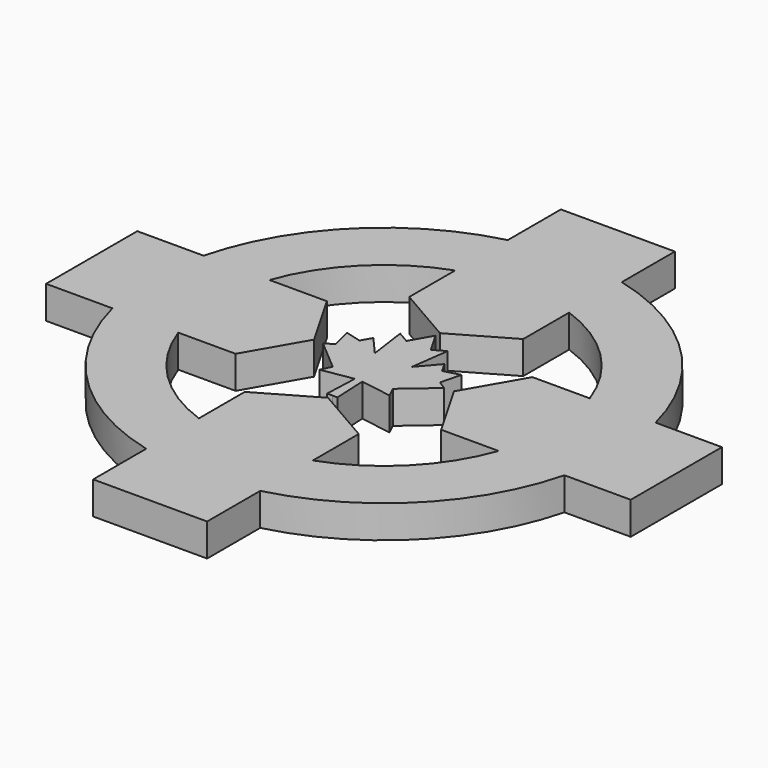
from build123d import *

# Parameters (mm, degrees)
F1_DEPTH = 5


with BuildPart() as f1:
    # F0 (on Top) → F1 (new body)
    with BuildSketch(Plane.XY):
        with BuildLine():
            Line((-8.7284976617, 44.7745621204), (-8.7284976617, 34.6139920432))
            ThreePointArc((-8.7284976617, 34.6139920432), (-4.3977485861, 35.4256252446), (0, 35.6975505686))
            Line((0, 35.6975505686), (0, 44.7745621204))
            Line((0, 44.7745621204), (-8.7284976617, 44.7745621204))
        make_face()
        with BuildLine():
            Line((0, 44.7745621204), (0, 35.6975505686))
            ThreePointArc((0, 35.6975505686), (4.3977485861, 35.4256252446), (8.7284976617, 34.6139920432))
            Line((8.7284976617, 34.6139920432), (8.7284976617, 44.7745621204))
            Line((8.7284976617, 44.7745621204), (0, 44.7745621204))
        make_face()
        with BuildLine():
            ThreePointArc((8.7284976617, 34.6139920432), (4.3977485861, 35.4256252446), (0, 35.6975505686))
            Line((0, 35.6975505686), (0, 26.0385947902))
            ThreePointArc((0, 26.0385947902), (4.4287789528, 25.6591959273), (8.7284976616, 24.5320555033))
            Line((8.7284976617, 24.5320555033), (8.7284976617, 34.6139920432))
        make_face()
        with BuildLine():
            ThreePointArc((0, 35.6975505686), (-4.3977485861, 35.4256252446), (-8.7284976617, 34.6139920432))
            Line((-8.7284976617, 34.6139920432), (-8.7284976617, 24.5320555033))
            ThreePointArc((-8.7284976616, 24.5320555033), (-4.4287789528, 25.6591959273), (0, 26.0385947902))
            Line((0, 26.0385947902), (0, 35.6975505686))
        make_face()
        with BuildLine():
            ThreePointArc((0, 26.0385947902), (-4.4287789528, 25.6591959273), (-8.7284976616, 24.5320555033))
            Line((-8.7284976617, 24.5320555033), (-8.7284976617, 15.7472789288))
            Line((-8.7284976617, 15.7472789288), (0, 10.7151791453))
            Line((0, 10.7151791453), (0, 26.0385947902))
        make_face()
        with BuildLine():
            ThreePointArc((8.7284976616, 24.5320555033), (4.4287789528, 25.6591959273), (0, 26.0385947902))
            Line((0, 26.0385947902), (0, 10.7151791453))
            Line((0, 10.7151791453), (8.7284976617, 15.7472789288))
            Line((8.7284976617, 15.7472789288), (8.7284976617, 24.5320555033))
        make_face()
        with BuildLine():
            Line((15.7472789288, -8.7284976617), (24.5320555033, -8.7284976617))
            ThreePointArc((24.5320555033, -8.7284976617), (25.6591959273, -4.4287789528), (26.0385947902, 0))
            Line((26.0385947902, 0), (10.7151791453, 0))
            Line((10.7151791453, 0), (15.7472789288, -8.7284976617))
        make_face()
        with BuildLine():
            ThreePointArc((26.0385947902, 0), (25.6591959273, 4.4287789528), (24.5320555033, 8.7284976616))
            Line((24.5320555033, 8.7284976617), (15.7472789288, 8.7284976617))
            Line((15.7472789288, 8.7284976617), (10.7151791453, 0))
            Line((10.7151791453, 0), (26.0385947902, 0))
        make_face()
        with BuildLine():
            ThreePointArc((35.6975505686, 0), (35.4256252446, 4.3977485861), (34.6139920432, 8.7284976616))
            Line((34.6139920432, 8.7284976617), (24.5320555033, 8.7284976617))
            ThreePointArc((24.5320555033, 8.7284976616), (25.6591959273, 4.4287789528), (26.0385947902, 0))
            Line((26.0385947902, 0), (35.6975505686, 0))
        make_face()
        with BuildLine():
            Line((24.5320555033, -8.7284976617), (34.6139920432, -8.7284976617))
            ThreePointArc((34.6139920432, -8.7284976616), (35.4256252446, -4.3977485861), (35.6975505686, 0))
            Line((35.6975505686, 0), (26.0385947902, 0))
            ThreePointArc((26.0385947902, 0), (25.6591959273, -4.4287789528), (24.5320555033, -8.7284976617))
        make_face()
        with BuildLine():
            ThreePointArc((35.6975505686, 0), (35.4256252446, -4.3977485861), (34.6139920432, -8.7284976616))
            Line((34.6139920432, -8.7284976617), (44.7745621204, -8.7284976617))
            Line((44.7745621204, -8.7284976617), (44.7745621204, 0))
            Line((44.7745621204, 0), (35.6975505686, 0))
        make_face()
        with BuildLine():
            Line((44.7745621204, 8.7284976617), (34.6139920432, 8.7284976617))
            ThreePointArc((34.6139920432, 8.7284976616), (35.4256252446, 4.3977485861), (35.6975505686, 0))
            Line((35.6975505686, 0), (44.7745621204, 0))
            Line((44.7745621204, 0), (44.7745621204, 8.7284976617))
        make_face()
        with BuildLine():
            ThreePointArc((34.6139920432, 8.7284976616), (25.2419800788, 25.2419800788), (8.7284976617, 34.6139920432))
            Line((8.7284976617, 34.6139920432), (8.7284976617, 24.5320555033))
            ThreePointArc((8.7284976616, 24.5320555033), (18.4120669487, 18.4120669487), (24.5320555033, 8.7284976616))
            Line((24.5320555033, 8.7284976617), (34.6139920432, 8.7284976617))
        make_face()
        with BuildLine():
            ThreePointArc((-8.7284976617, 34.6139920432), (-25.2419800788, 25.2419800788), (-34.6139920432, 8.7284976616))
            Line((-34.6139920432, 8.7284976617), (-24.5320555033, 8.7284976617))
            ThreePointArc((-24.5320555033, 8.7284976616), (-18.4120669487, 18.4120669487), (-8.7284976616, 24.5320555033))
            Line((-8.7284976617, 24.5320555033), (-8.7284976617, 34.6139920432))
        make_face()
        with BuildLine():
            ThreePointArc((-34.6139920432, 8.7284976616), (-35.4256252446, 4.3977485861), (-35.6975505686, 0))
            Line((-35.6975505686, 0), (-26.0385947902, 0))
            ThreePointArc((-26.0385947902, 0), (-25.6591959273, 4.4287789528), (-24.5320555033, 8.7284976616))
            Line((-24.5320555033, 8.7284976617), (-34.6139920432, 8.7284976617))
        make_face()
        with BuildLine():
            ThreePointArc((-24.5320555033, 8.7284976616), (-25.6591959273, 4.4287789528), (-26.0385947902, 0))
            Line((-26.0385947902, 0), (-10.7151791453, 0))
            Line((-10.7151791453, 0), (-15.7472789288, 8.7284976617))
            Line((-15.7472789288, 8.7284976617), (-24.5320555033, 8.7284976617))
        make_face()
        with BuildLine():
            Line((-10.7151791453, 0), (-26.0385947902, 0))
            ThreePointArc((-26.0385947902, 0), (-25.6591959273, -4.4287789528), (-24.5320555033, -8.7284976616))
            Line((-24.5320555033, -8.7284976617), (-15.7472789288, -8.7284976617))
            Line((-15.7472789288, -8.7284976617), (-10.7151791453, 0))
        make_face()
        with BuildLine():
            Line((-26.0385947902, 0), (-35.6975505686, 0))
            ThreePointArc((-35.6975505686, 0), (-35.4256252446, -4.3977485861), (-34.6139920432, -8.7284976616))
            Line((-34.6139920432, -8.7284976617), (-24.5320555033, -8.7284976617))
            ThreePointArc((-24.5320555033, -8.7284976616), (-25.6591959273, -4.4287789528), (-26.0385947902, 0))
        make_face()
        with BuildLine():
            Line((-35.6975505686, 0), (-44.7745621204, 0))
            Line((-44.7745621204, 0), (-44.7745621204, -8.7284976617))
            Line((-44.7745621204, -8.7284976617), (-34.6139920432, -8.7284976617))
            ThreePointArc((-34.6139920432, -8.7284976616), (-35.4256252446, -4.3977485861), (-35.6975505686, 0))
        make_face()
        with BuildLine():
            Line((-44.7745621204, 8.7284976617), (-44.7745621204, 0))
            Line((-44.7745621204, 0), (-35.6975505686, 0))
            ThreePointArc((-35.6975505686, 0), (-35.4256252446, 4.3977485861), (-34.6139920432, 8.7284976616))
            Line((-34.6139920432, 8.7284976617), (-44.7745621204, 8.7284976617))
        make_face()
        with BuildLine():
            Line((-24.5320555033, -8.7284976617), (-34.6139920432, -8.7284976617))
            ThreePointArc((-34.6139920432, -8.7284976616), (-25.2419800788, -25.2419800788), (-8.7284976617, -34.6139920432))
            Line((-8.7284976617, -34.6139920432), (-8.7284976617, -24.5320555033))
            ThreePointArc((-8.7284976616, -24.5320555033), (-18.4120669487, -18.4120669487), (-24.5320555033, -8.7284976616))
        make_face()
        with BuildLine():
            Line((-8.7284976617, -24.5320555033), (-8.7284976617, -34.6139920432))
            ThreePointArc((-8.7284976617, -34.6139920432), (-4.3977485861, -35.4256252446), (0, -35.6975505686))
            Line((0, -35.6975505686), (0, -26.0385947902))
            ThreePointArc((0, -26.0385947902), (-4.4287789528, -25.6591959273), (-8.7284976616, -24.5320555033))
        make_face()
        with BuildLine():
            Line((-8.7284976617, -15.7472789288), (-8.7284976617, -24.5320555033))
            ThreePointArc((-8.7284976616, -24.5320555033), (-4.4287789528, -25.6591959273), (0, -26.0385947902))
            Line((0, -26.0385947902), (0, -10.7151791453))
            Line((0, -10.7151791453), (-8.7284976617, -15.7472789288))
        make_face()
        with BuildLine():
            Line((0, -10.7151791453), (0, -26.0385947902))
            ThreePointArc((0, -26.0385947902), (4.4287789528, -25.6591959273), (8.7284976616, -24.5320555033))
            Line((8.7284976617, -24.5320555033), (8.7284976617, -15.7472789288))
            Line((8.7284976617, -15.7472789288), (0, -10.7151791453))
        make_face()
        with BuildLine():
            Line((0, -26.0385947902), (0, -35.6975505686))
            ThreePointArc((0, -35.6975505686), (4.3977485861, -35.4256252446), (8.7284976617, -34.6139920432))
            Line((8.7284976617, -34.6139920432), (8.7284976617, -24.5320555033))
            ThreePointArc((8.7284976616, -24.5320555033), (4.4287789528, -25.6591959273), (0, -26.0385947902))
        make_face()
        with BuildLine():
            Line((8.7284976617, -24.5320555033), (8.7284976617, -34.6139920432))
            ThreePointArc((8.7284976617, -34.6139920432), (25.2419800788, -25.2419800788), (34.6139920432, -8.7284976616))
            Line((34.6139920432, -8.7284976617), (24.5320555033, -8.7284976617))
            ThreePointArc((24.5320555033, -8.7284976617), (18.4120669487, -18.4120669487), (8.7284976616, -24.5320555033))
        make_face()
        with BuildLine():
            ThreePointArc((8.7284976617, -34.6139920432), (4.3977485861, -35.4256252446), (0, -35.6975505686))
            Line((0, -35.6975505686), (0, -44.7745621204))
            Line((0, -44.7745621204), (8.7284976617, -44.7745621204))
            Line((8.7284976617, -44.7745621204), (8.7284976617, -34.6139920432))
        make_face()
        with BuildLine():
            ThreePointArc((0, -35.6975505686), (-4.3977485861, -35.4256252446), (-8.7284976617, -34.6139920432))
            Line((-8.7284976617, -34.6139920432), (-8.7284976617, -44.7745621204))
            Line((-8.7284976617, -44.7745621204), (0, -44.7745621204))
            Line((0, -44.7745621204), (0, -35.6975505686))
        make_face()
    extrude(amount=F1_DEPTH)


with BuildPart() as f1b:
    # F0 (on Top) → F1, piece 2 (new body)
    with BuildSketch(Plane.XY):
        Polygon((0.0193861542, -9.910623543), (0, 0), (0, 9.8333135078), (-0.019299824, 9.8664896445), (-1.8821764336, 6.6352114842), (-3.652818574, 7.6560111999), (-2.8409659863, 1.7956340453), (-5.4364711978, 4.7619254328), (-6.3354833617, 3.2025315598), (-8.7735494599, 3.8614440709), (-7.9790065065, 0.7362440811), (-9.2502748594, -0.1112677855), (-4.588959273, -4.0839798748), (-5.3305323236, -5.6730648503), (-0.5632776883, -4.8785223626), (-0.7751554949, -9.9635934457), align=None)
        Polygon((0, 9.8333135078), (0, 0), (0.0193861542, -9.910623543), (0.814128951, -9.9604846491), (0.5823590437, -4.8762813845), (5.3526855916, -5.6521674255), (4.6049014268, -4.0659957792), (9.2506393704, -0.075078178), (7.9760651256, 0.7674537701), (8.7583756485, 3.8957382405), (6.3229059933, 3.2272926142), (5.417800077, 4.7831574548), (2.8339193988, 1.8067346791), (3.6228389134, 7.6702431014), (1.856203877, 6.6425241237), align=None)
    extrude(amount=F1_DEPTH)


solid = Compound([f1.part, f1b.part])
